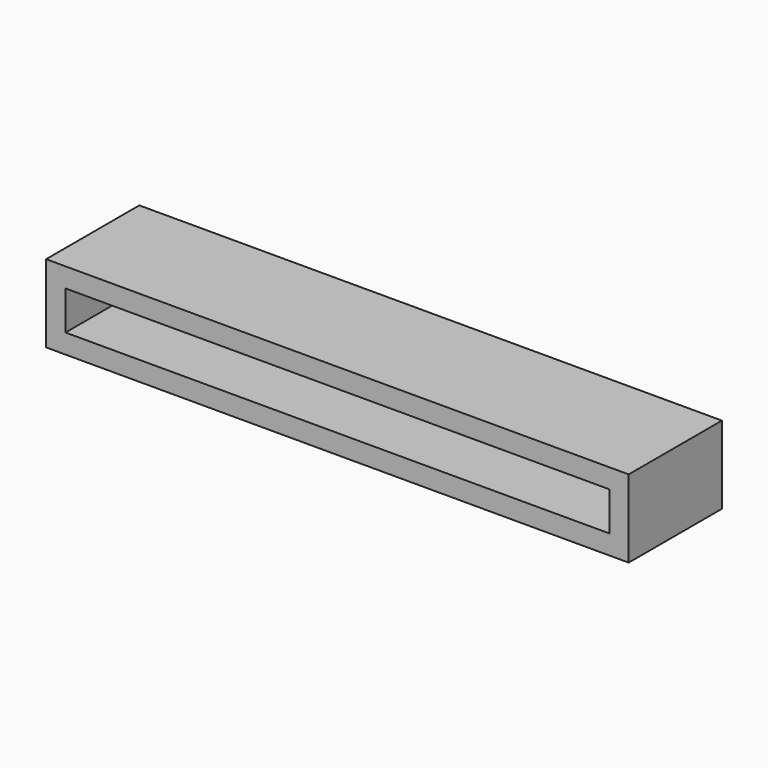
from build123d import *

# Parameters (mm, degrees)
F0_W     = 38.1
F0_H     = 5.08
F1_DEPTH = 7.62
F3_T     = -1.27


# Not quite as in the source:
# - a feature of the source that left no trace in its solid (it failed there, or was rolled back) is left out


with BuildPart() as f1:
    # F0 (on Front) → F1 (new body)
    with BuildSketch(Plane.XZ):
        with Locations((-46.2881572708, 42.3315375688)):
            Rectangle(F0_W, F0_H)
    extrude(amount=F1_DEPTH)

    # F3
    f3_openings = [f1.faces().sort_by_distance(p)[0] for p in [
        (-46.288157, -7.62, 42.331538),
    ]]
    offset(amount=F3_T, openings=f3_openings)


solid = f1.part
